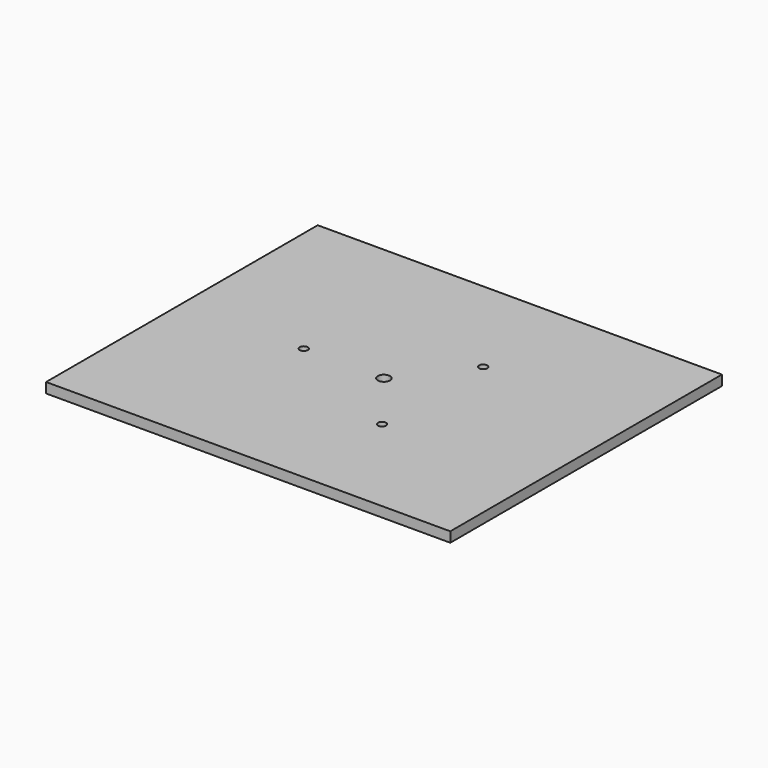
from build123d import *

# Parameters (mm, degrees)
F0_W     = 317.5
F0_H     = 266.7
F0_R     = 3.175
F0_R_2   = 4.7625
F1_DEPTH = 7.9375


# Not quite as in the source:
# - a feature names something its author has since deleted; it is built from what else it names


with BuildPart() as f1:
    # F0 (on Top) → F1 (new body)
    with BuildSketch(Plane.XY):
        with Locations((0.0623334384, 0.0151203394)):
            Rectangle(F0_W, F0_H)
        with Locations((-62.9493173903, -0.0005464993)):
            Circle(F0_R, mode=Mode.SUBTRACT)
        Circle(F0_R_2, mode=Mode.SUBTRACT)
        with Locations((37.2055072098, -48.3364977443)):
            Circle(F0_R, mode=Mode.SUBTRACT)
        with Locations((38.0921348072, 49.8540893279)):
            Circle(F0_R, mode=Mode.SUBTRACT)
    extrude(amount=F1_DEPTH)


solid = f1.part
